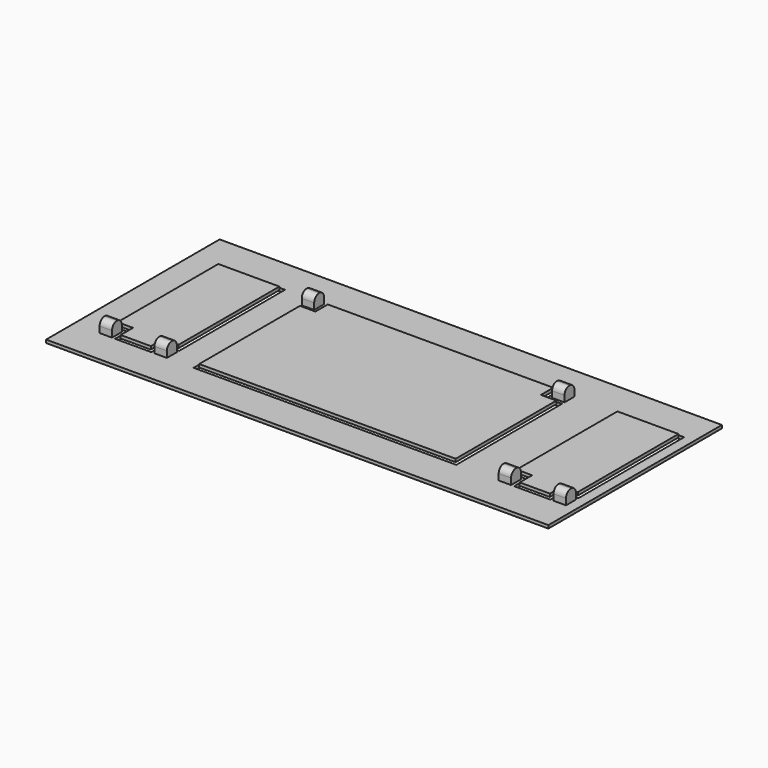
from build123d import *

# Parameters (mm, degrees)
F0_W     = 162.2753325211
F0_H     = 70.084847109
F0_W_2   = 4
F0_H_2   = 4
F1_DEPTH = 1
F2_DEPTH = 4
F3_R     = 1.99999
F4_DEPTH = 1


# Not quite as in the source:
# - a fillet or chamfer is up to 0.001 mm smaller than in the source, because OpenCascade refuses the exact size


with BuildPart() as f1:
    # F0 (on Top) → F1 (new body)
    with BuildSketch(Plane.XY):
        with Locations((0, 1.7718460756)):
            Rectangle(F0_W, F0_H)
        with Locations((-70.8014665545, -20.0708878118)):
            Rectangle(F0_W_2, F0_H_2, mode=Mode.SUBTRACT)
        with Locations((-53.0607582087, -20.0708878118)):
            Rectangle(F0_W_2, F0_H_2, mode=Mode.SUBTRACT)
        Polygon((-72.8014665545, -17.0708878118), (-72.8014665545, 25.6145799629), (-51.0607582087, 25.6145799629), (-51.0607582087, -17.0708878118), (-56.0607582087, -17.0708878118), (-56.0607582087, -22.0708878118), (-67.8014665545, -22.0708878118), (-67.8014665545, -17.0708878118), align=None, mode=Mode.SUBTRACT)
        with Locations((58.1299888442, -20.0708878118)):
            Rectangle(F0_W_2, F0_H_2, mode=Mode.SUBTRACT)
        with Locations((75.87069719, -20.0708878118)):
            Rectangle(F0_W_2, F0_H_2, mode=Mode.SUBTRACT)
        with Locations((-40.4279221569, 23.6145799629)):
            Rectangle(F0_W_2, F0_H_2, mode=Mode.SUBTRACT)
        Polygon((-37.4279221569, 20.6145799629), (-37.4279221569, 25.6145799629), (37.4279221569, 25.6145799629), (37.4279221569, 20.6145799629), (42.4279221569, 20.6145799629), (42.4279221569, -22.0708878118), (-42.4279221569, -22.0708878118), (-42.4279221569, 20.6145799629), align=None, mode=Mode.SUBTRACT)
        with Locations((40.4279221569, 23.6145799629)):
            Rectangle(F0_W_2, F0_H_2, mode=Mode.SUBTRACT)
        Polygon((72.87069719, -17.0708878118), (72.87069719, -22.0708878118), (61.1299888442, -22.0708878118), (61.1299888442, -17.0708878118), (56.1299888442, -17.0708878118), (56.1299888442, 25.6145799629), (77.87069719, 25.6145799629), (77.87069719, -17.0708878118), align=None, mode=Mode.SUBTRACT)
        with Locations((-53.0607582087, -20.0708878118)):
            Rectangle(F0_W_2, F0_H_2)
        with Locations((-70.8014665545, -20.0708878118)):
            Rectangle(F0_W_2, F0_H_2)
        with Locations((40.4279221569, 23.6145799629)):
            Rectangle(F0_W_2, F0_H_2)
        with Locations((-40.4279221569, 23.6145799629)):
            Rectangle(F0_W_2, F0_H_2)
        with Locations((75.87069719, -20.0708878118)):
            Rectangle(F0_W_2, F0_H_2)
        with Locations((58.1299888442, -20.0708878118)):
            Rectangle(F0_W_2, F0_H_2)
    extrude(amount=-F1_DEPTH)

    # F0 (on Top) → F2 (join)
    with BuildSketch(Plane.XY):
        with Locations((-70.8014665545, -20.0708878118)):
            Rectangle(F0_W_2, F0_H_2)
        with Locations((-53.0607582087, -20.0708878118)):
            Rectangle(F0_W_2, F0_H_2)
        with Locations((-40.4279221569, 23.6145799629)):
            Rectangle(F0_W_2, F0_H_2)
        with Locations((40.4279221569, 23.6145799629)):
            Rectangle(F0_W_2, F0_H_2)
        with Locations((75.87069719, -20.0708878118)):
            Rectangle(F0_W_2, F0_H_2)
        with Locations((58.1299888442, -20.0708878118)):
            Rectangle(F0_W_2, F0_H_2)
    extrude(amount=F2_DEPTH)

    # F3 (radius 2 in the source; OpenCascade refuses exactly that, so slightly less here)
    f3_edges = [f1.edges().sort_by_distance(p)[0] for p in [
        (-70.801467, -18.070888, 4),
        (-70.801467, -22.070888, 4),
        (-53.060758, -18.070888, 4),
        (-53.060758, -22.070888, 4),
        (-40.427922, 25.61458, 4),
        (-40.427922, 21.61458, 4),
        (40.427922, 25.61458, 4),
        (40.427922, 21.61458, 4),
        (58.129989, -18.070888, 4),
        (58.129989, -22.070888, 4),
        (75.870697, -22.070888, 4),
        (75.870697, -18.070888, 4),
    ]]
    fillet(f3_edges, radius=F3_R)


with BuildPart() as f4:
    # F0 (on Top) → F4 (new body)
    with BuildSketch(Plane.XY):
        Polygon((-52.0607582087, -16.0708878118), (-52.0607582087, 24.6145799629), (-71.8014665545, 24.6145799629), (-71.8014665545, -16.0708878118), (-66.8014665545, -16.0708878118), (-66.8014665545, -21.0708878118), (-57.0607582087, -21.0708878118), (-57.0607582087, -16.0708878118), align=None)
    extrude(amount=F4_DEPTH)


with BuildPart() as f4b:
    # F0 (on Top) → F4, piece 2 (new body)
    with BuildSketch(Plane.XY):
        Polygon((-36.4279221569, 19.6145799629), (-41.4279221569, 19.6145799629), (-41.4279221569, -21.0708878118), (41.4279221569, -21.0708878118), (41.4279221569, 19.6145799629), (36.4279221569, 19.6145799629), (36.4279221569, 24.6145799629), (-36.4279221569, 24.6145799629), align=None)
    extrude(amount=F4_DEPTH)


with BuildPart() as f4c:
    # F0 (on Top) → F4, piece 3 (new body)
    with BuildSketch(Plane.XY):
        Polygon((76.87069719, -16.0708878118), (76.87069719, 24.6145799629), (57.1299888442, 24.6145799629), (57.1299888442, -16.0708878118), (62.1299888442, -16.0708878118), (62.1299888442, -21.0708878118), (71.87069719, -21.0708878118), (71.87069719, -16.0708878118), align=None)
    extrude(amount=F4_DEPTH)


solid = Compound([f1.part, f4.part, f4b.part, f4c.part])
